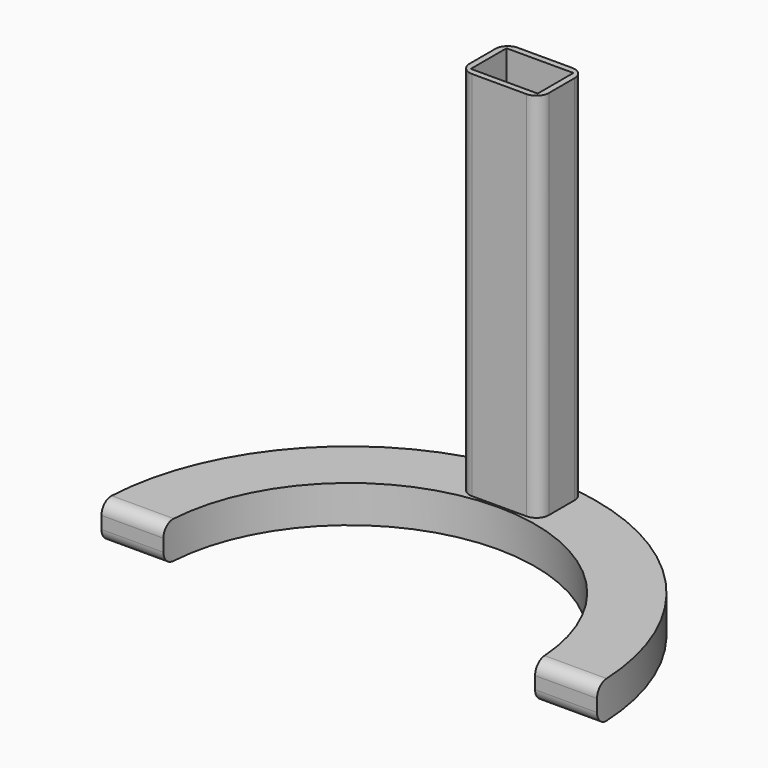
from build123d import *

# Parameters (mm, degrees)
F1_DEPTH    = 15
F2_W        = 32
F2_H        = 23
F3_DEPTH    = 150
F4_T        = 2.5
F4_T3_DEPTH = 28
F4_T5_DEPTH = 37
F5_R        = 5


# Not quite as in the source:
# - a shell that OpenCascade refuses in one call is made with other operations: the cavity is built on its own and cut out


with BuildPart() as f1:
    # F0 (on Top) → F1 (new body)
    with BuildSketch(Plane.XY):
        with BuildLine():
            Line((75, 0), (100, 0))
            ThreePointArc((100, 0), (0, 100), (-100, 0))
            Line((-100, 0), (-75, 0))
            ThreePointArc((-75, 0), (0, 75), (75, 0))
        make_face()
    extrude(amount=F1_DEPTH)

    # F2 (on face) → F3 (join)
    with BuildSketch(Plane.XY.offset(15)):
        with Locations((0, 87.211701434)):
            Rectangle(F2_W, F2_H)
    extrude(amount=F3_DEPTH)

    # F4: shell of thickness 2.5, made by hand


with BuildPart() as f4_core1:
    # F4_t2: copy of F1
    add(f1.part)

    # the walls: a layer under each face that stays
    f4_faces = [f4_core1.faces().sort_by_distance(p)[0] for p in [
        (-87.5, 0, 7.5),
        (0, 100, 7.5),
        (0, 75, 7.5),
        (-66.6666666667, 50, 0),
        (-66.6666666667, 49.355850717, 15),
        (87.5, 0, 7.5),
        (0, 99.355850717, 15),
        (-16, 87.211701434, 90),
        (0, 75.711701434, 90),
        (16, 87.211701434, 90),
        (0, 98.711701434, 90),
    ]]
    thicken(f4_faces, amount=-F4_T, mode=Mode.SUBTRACT)

    # F4_s4 → F4_t3 (cut)
    with BuildSketch(Plane.XZ.offset(-101.211701434)):
        Polygon((-16.025, 15.025), (-16, 12.5), (-13.5, 12.5), (-13.5, 15), align=None)
        Polygon((16.025, 15.025), (16, 12.5), (13.5, 12.5), (13.5, 15), align=None)
    extrude(amount=F4_T3_DEPTH, mode=Mode.SUBTRACT)

    # F4_s6 → F4_t5 (cut)
    with BuildSketch(Plane.YZ.offset(-18.5)):
        Polygon((75.686701434, 15.025), (75.711701434, 12.5), (78.211701434, 12.5), (78.211701434, 15), align=None)
        Polygon((98.736701434, 15.025), (98.711701434, 12.5), (96.211701434, 12.5), (96.211701434, 15), align=None)
    extrude(amount=F4_T5_DEPTH, mode=Mode.SUBTRACT)


with BuildPart() as f1_1:
    add(f1.part)

    # what is left inside the walls is the cavity
    f4_cavity = [f4_core1.part.solids().sort_by_distance(p)[0] for p in [
        (-48.733972, 65.833333, 2.525),
    ]]
    add(f4_cavity, mode=Mode.SUBTRACT)

    # F5
    f5_edges = [f1_1.edges().sort_by_distance(p)[0] for p in [
        (-16, 75.711701, 90),
        (-16, 98.711701, 90),
        (16, 98.711701, 90),
        (16, 75.711701, 90),
        (-87.5, 0, 15),
        (-87.5, 0, 0),
        (87.5, 0, 15),
        (87.5, 0, 0),
    ]]
    fillet(f5_edges, radius=F5_R)


solid = f1_1.part
